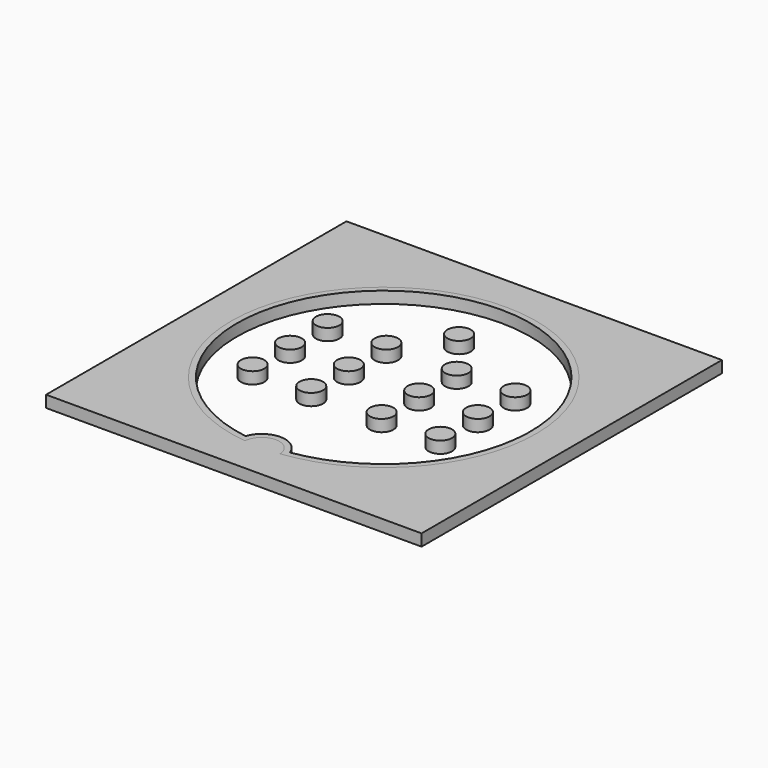
from build123d import *

# Parameters (mm, degrees)
F1_DEPTH = 1
F0_R     = 1
F0_W     = 32
F0_H     = 32
F2_DEPTH = 1


# Not quite as in the source:
# - a feature names something its author has since deleted; it is built from what else it names


with BuildPart() as f1:
    # F0 (on Top) → F1 (new body)
    with BuildSketch(Plane.XY):
        with BuildLine():
            ThreePointArc((-1.5110484064, -12.9270083272), (-0.0135467888, -11.5135467888), (1.4839548288, -12.9270083272))
            ThreePointArc((1.4839548288, -12.9270083272), (-0.0135467888, 12.9864532112), (-1.5110484064, -12.9270083272))
        make_face()
        with BuildLine():
            ThreePointArc((-1.9069476222, -12.3693160195), (-0.0135467888, 12.4864532112), (1.8798540446, -12.3693160195))
            ThreePointArc((1.8798540446, -12.3693160195), (-0.0135467888, -11.0135467888), (-1.9069476222, -12.3693160195))
        make_face(mode=Mode.SUBTRACT)
    extrude(amount=F1_DEPTH)


with BuildPart() as f1b:
    # F0 (on Top) → F1, piece 2 (new body)
    with BuildSketch(Plane.XY):
        with Locations((-8, 4)):
            Circle(F0_R)
    extrude(amount=F1_DEPTH)


with BuildPart() as f1c:
    # F0 (on Top) → F1, piece 3 (new body)
    with BuildSketch(Plane.XY):
        with Locations((-3, 4)):
            Circle(F0_R)
    extrude(amount=F1_DEPTH)


with BuildPart() as f1d:
    # F0 (on Top) → F1, piece 4 (new body)
    with BuildSketch(Plane.XY):
        with Locations((0, 8)):
            Circle(F0_R)
    extrude(amount=F1_DEPTH)


with BuildPart() as f1e:
    # F0 (on Top) → F1, piece 5 (new body)
    with BuildSketch(Plane.XY):
        with Locations((3, 4)):
            Circle(F0_R)
    extrude(amount=F1_DEPTH)


with BuildPart() as f1f:
    # F0 (on Top) → F1, piece 6 (new body)
    with BuildSketch(Plane.XY):
        with Locations((8, 4)):
            Circle(F0_R)
    extrude(amount=F1_DEPTH)


with BuildPart() as f1g:
    # F0 (on Top) → F1, piece 7 (new body)
    with BuildSketch(Plane.XY):
        with Locations((8, 0)):
            Circle(F0_R)
    extrude(amount=F1_DEPTH)


with BuildPart() as f1h:
    # F0 (on Top) → F1, piece 8 (new body)
    with BuildSketch(Plane.XY):
        with Locations((8, -4)):
            Circle(F0_R)
    extrude(amount=F1_DEPTH)


with BuildPart() as f1i:
    # F0 (on Top) → F1, piece 9 (new body)
    with BuildSketch(Plane.XY):
        with Locations((3, -4)):
            Circle(F0_R)
    extrude(amount=F1_DEPTH)


with BuildPart() as f1j:
    # F0 (on Top) → F1, piece 10 (new body)
    with BuildSketch(Plane.XY):
        with Locations((3, 0)):
            Circle(F0_R)
    extrude(amount=F1_DEPTH)


with BuildPart() as f1k:
    # F0 (on Top) → F1, piece 11 (new body)
    with BuildSketch(Plane.XY):
        with Locations((-3, 0)):
            Circle(F0_R)
    extrude(amount=F1_DEPTH)


with BuildPart() as f1l:
    # F0 (on Top) → F1, piece 12 (new body)
    with BuildSketch(Plane.XY):
        with Locations((-3, -4)):
            Circle(F0_R)
    extrude(amount=F1_DEPTH)


with BuildPart() as f1m:
    # F0 (on Top) → F1, piece 13 (new body)
    with BuildSketch(Plane.XY):
        with Locations((-8, -4)):
            Circle(F0_R)
    extrude(amount=F1_DEPTH)


with BuildPart() as f1n:
    # F0 (on Top) → F1, piece 14 (new body)
    with BuildSketch(Plane.XY):
        with Locations((-8, 0)):
            Circle(F0_R)
    extrude(amount=F1_DEPTH)


with BuildPart() as f2:
    # F0 (on Top) → F2 (new body)
    with BuildSketch(Plane.XY):
        Rectangle(F0_W, F0_H)
        with BuildLine():
            ThreePointArc((-1.5110484064, -12.9270083272), (-0.0135467888, 12.9864532112), (1.4839548288, -12.9270083272))
            ThreePointArc((1.4839548288, -12.9270083272), (-0.0135467888, -11.5135467888), (-1.5110484064, -12.9270083272))
        make_face(mode=Mode.SUBTRACT)
    extrude(amount=F2_DEPTH)


solid = Compound([f1.part, f1b.part, f1c.part, f1d.part, f1e.part, f1f.part, f1g.part, f1h.part, f1i.part, f1j.part, f1k.part, f1l.part, f1m.part, f1n.part, f2.part])
